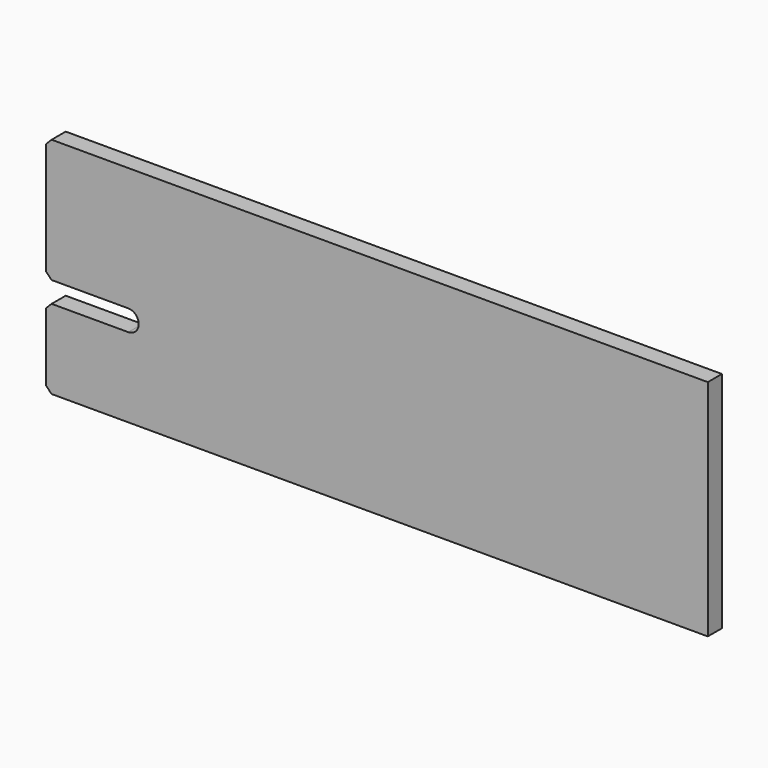
from build123d import *

# Parameters (mm, degrees)
F0_W     = 60
F0_H     = 20.3
F1_DEPTH = 1.6
F2_W     = 10
F2_H     = 1.9
F3_DEPTH = 25
F4_SIZE  = 0.5
F5_R     = 0.94999


# Not quite as in the source:
# - a fillet or chamfer is up to 0.001 mm smaller than in the source, because OpenCascade refuses the exact size


with BuildPart() as f1:
    # F0 (on Front) → F1 (new body)
    with BuildSketch(Plane.XZ):
        with Locations((19.8222492922, -0.2282736823)):
            Rectangle(F0_W, F0_H)
    extrude(amount=F1_DEPTH)

    # F2 (on Front) → F3 (cut)
    with BuildSketch(Plane.XZ):
        with Locations((-6.7777507078, -2.2282736823)):
            Rectangle(F2_W, F2_H)
    extrude(amount=F3_DEPTH, mode=Mode.SUBTRACT)

    # F4
    f4_edges = [f1.edges().sort_by_distance(p)[0] for p in [
        (-10.177751, -0.8, 9.921726),
        (-10.177751, -0.8, -1.278274),
        (-10.177751, -0.8, -3.178274),
        (-10.177751, -0.8, -10.378274),
    ]]
    chamfer(f4_edges, length=F4_SIZE)

    # F5 (radius 0.95 in the source; OpenCascade refuses exactly that, so slightly less here)
    f5_edges = [f1.edges().sort_by_distance(p)[0] for p in [
        (-1.777751, -0.8, -1.278274),
        (-1.777751, -0.8, -3.178274),
    ]]
    fillet(f5_edges, radius=F5_R)


solid = f1.part
